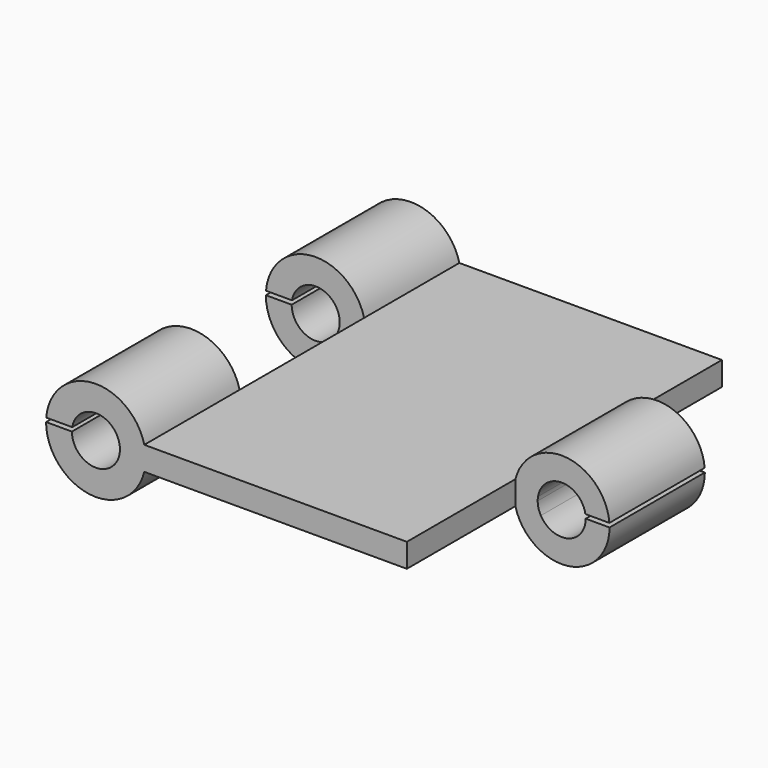
from build123d import *

# Parameters (mm, degrees)
F1_DEPTH = 87.2
F2_DEPTH = 12
F4_W     = 36.556558
F4_H     = 39.2
F5_DEPTH = 112.6


with BuildPart() as f1:
    # F0 (on Front) → F1 (new body)
    with BuildSketch(Plane.XZ):
        with BuildLine():
            ThreePointArc((-55.908021, 8.682486), (-51.001267, 13.638898), (-44.685806, 10.67964))
            Line((-44.685806, 10.67964), (-37.754378, 10.67964))
            ThreePointArc((-37.754378, 10.67964), (-50.952809, 20.191652), (-62.451334, 8.682486))
            Line((-62.451334, 8.682486), (-55.908021, 8.682486))
        make_face()
        with BuildLine():
            Line((-37.75418, 4.686138), (-44.685347, 4.686138))
            ThreePointArc((-44.685347, 4.686138), (-51.491134, 1.834382), (-55.991238, 7.682486))
            Line((-55.991238, 7.682486), (-62.491238, 7.682486))
            ThreePointArc((-62.491238, 7.682486), (-51.450363, -4.776448), (-37.75418, 4.686138))
        make_face()
        with BuildLine():
            Line((28.008762, 7.682486), (-37.391238, 7.682486))
            ThreePointArc((-37.391238, 7.682486), (-37.482304, 6.173362), (-37.75418, 4.686138))
            Line((-37.75418, 4.686138), (28.387241, 4.686138))
            ThreePointArc((28.387241, 4.686138), (28.103756, 6.172408), (28.008762, 7.682486))
        make_face()
        with BuildLine():
            ThreePointArc((52.067196, 8.682486), (41.071465, 19.689856), (28.387448, 10.67964))
            Line((28.387448, 10.67964), (34.803329, 10.67964))
            ThreePointArc((34.803329, 10.67964), (41.11879, 13.638898), (46.025545, 8.682486))
            Line((46.025545, 8.682486), (52.067196, 8.682486))
        make_face()
        with BuildLine():
            Line((34.80287, 4.686138), (28.387241, 4.686138))
            ThreePointArc((28.387241, 4.686138), (41.56884, -4.272519), (52.108762, 7.682486))
            Line((52.108762, 7.682486), (46.108762, 7.682486))
            ThreePointArc((46.108762, 7.682486), (41.608658, 1.834382), (34.80287, 4.686138))
        make_face()
        with BuildLine():
            ThreePointArc((-37.754378, 10.67964), (-37.55245, 9.687587), (-37.431142, 8.682486))
            Line((-37.431142, 8.682486), (28.050327, 8.682486))
            ThreePointArc((28.050327, 8.682486), (28.176852, 9.688159), (28.387448, 10.67964))
            Line((28.387448, 10.67964), (-37.754378, 10.67964))
        make_face()
        with BuildLine():
            ThreePointArc((-44.685806, 10.67964), (-44.241968, 9.712465), (-43.974455, 8.682486))
            Line((-43.974455, 8.682486), (-37.431142, 8.682486))
            ThreePointArc((-37.431142, 8.682486), (-37.55245, 9.687587), (-37.754378, 10.67964))
            Line((-37.754378, 10.67964), (-44.685806, 10.67964))
        make_face()
        with BuildLine():
            Line((-37.391238, 7.682486), (-43.891238, 7.682486))
            ThreePointArc((-43.891238, 7.682486), (-44.093134, 6.13259), (-44.685347, 4.686138))
            Line((-44.685347, 4.686138), (-37.75418, 4.686138))
            ThreePointArc((-37.75418, 4.686138), (-37.482304, 6.173362), (-37.391238, 7.682486))
        make_face()
        with BuildLine():
            Line((34.008762, 7.682486), (28.008762, 7.682486))
            ThreePointArc((28.008762, 7.682486), (28.103756, 6.172408), (28.387241, 4.686138))
            Line((28.387241, 4.686138), (34.80287, 4.686138))
            ThreePointArc((34.80287, 4.686138), (34.210657, 6.13259), (34.008762, 7.682486))
        make_face()
        with BuildLine():
            ThreePointArc((28.387448, 10.67964), (28.176852, 9.688159), (28.050327, 8.682486))
            Line((28.050327, 8.682486), (34.091979, 8.682486))
            ThreePointArc((34.091979, 8.682486), (34.359491, 9.712465), (34.803329, 10.67964))
            Line((34.803329, 10.67964), (28.387448, 10.67964))
        make_face()
        with BuildLine():
            ThreePointArc((-37.431142, 8.682486), (-37.401218, 8.182884), (-37.391238, 7.682486))
            Line((-37.391238, 7.682486), (28.008762, 7.682486))
            ThreePointArc((28.008762, 7.682486), (28.019157, 8.182918), (28.050327, 8.682486))
            Line((28.050327, 8.682486), (-37.431142, 8.682486))
        make_face()
        with BuildLine():
            ThreePointArc((-43.974455, 8.682486), (-43.912079, 8.184215), (-43.891238, 7.682486))
            Line((-43.891238, 7.682486), (-37.391238, 7.682486))
            ThreePointArc((-37.391238, 7.682486), (-37.401218, 8.182884), (-37.431142, 8.682486))
            Line((-37.431142, 8.682486), (-43.974455, 8.682486))
        make_face()
        with BuildLine():
            ThreePointArc((28.050327, 8.682486), (28.019157, 8.182918), (28.008762, 7.682486))
            Line((28.008762, 7.682486), (34.008762, 7.682486))
            ThreePointArc((34.008762, 7.682486), (34.029602, 8.184215), (34.091979, 8.682486))
            Line((34.091979, 8.682486), (28.050327, 8.682486))
        make_face()
    extrude(amount=F1_DEPTH)

    # F2 (add): a face of the model
    f2_faces = [f1.faces().sort_by_distance(p)[0] for p in [
        (-6.403086, -87.2, 7.67694),
    ]]
    extrude(f2_faces, amount=F2_DEPTH)

    # F4 (on offset) → F5 (cut)
    with BuildSketch(Plane.XY.offset(35.67964)):
        Polygon((28.387448, -65.03436), (28.387448, -99.2), (28.387448, -157.014415), (88.272154, -157.014415), (88.272154, -65.03436), (66.477835, -65.03436), align=None)
        Polygon((28.387448, 0), (28.387448, -35.03436), (66.477835, -35.03436), (79.681844, -35.03436), (79.681844, 31.784113), (28.387448, 31.784113), align=None)
        with Locations((-56.032657, -49.6)):
            Rectangle(F4_W, F4_H)
    extrude(amount=-F5_DEPTH, mode=Mode.SUBTRACT)


solid = f1.part
